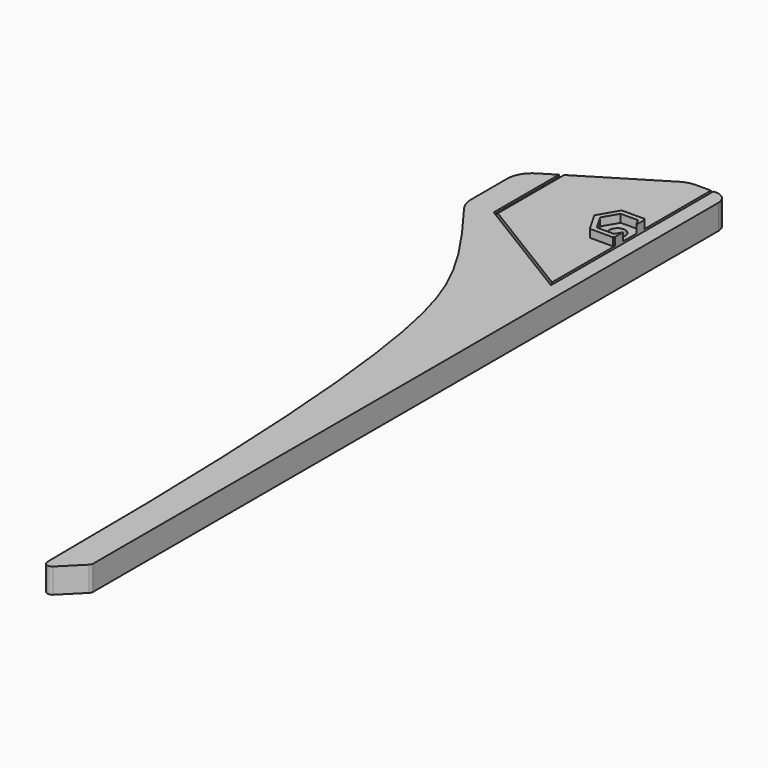
from build123d import *

# Parameters (mm, degrees)
F0_R        = 1.6
F1_DEPTH    = 2
F2_DEPTH    = 5
F3_START    = 2.1
F3_DEPTH    = 2.9
F4_SIZE     = 2.49999
F5_R        = 5
F6_R        = 2.5
F7_R        = 1
F8_START    = 2.1
F8_DEPTH    = 2.9
F9_T1_DEPTH = 29.797383518
F11_DEPTH   = 2.9
F12_DEPTH   = 4.5
F13_R       = 5


# Not quite as in the source:
# - a fillet or chamfer that OpenCascade refuses, or shapes differently, is made with other operations: its cross-section is extruded or revolved along the edge and cut away or added
# - a fillet or chamfer is up to 0.001 mm smaller than in the source, because OpenCascade refuses the exact size


with BuildPart() as f1:
    # F0 (on Top) → F1 (new body)
    with BuildSketch(Plane.XY):
        Polygon((1.5, 14.3055555556), (1.5, -2.088612395), (19, -12.7830568394), (24, -15.838612395), (24, 25), (19, 25), align=None)
        with Locations((21, 4.5806938025)):
            Circle(F0_R, mode=Mode.SUBTRACT)
        Polygon((-1, 12.7777777778), (-1, -0.5608346172), (1.5, -2.088612395), (1.5, 14.3055555556), align=None)
    extrude(amount=F1_DEPTH)

    # F0 (on Top) → F2 (join)
    with BuildSketch(Plane.XY):
        with BuildLine():
            Line((1.5, -2.088612395), (-1, -0.5608346172))
            Line((-1, -0.5608346172), (-1, 12.7777777778))
            Line((-1, 12.7777777778), (-4, 10.9444444444))
            Line((-4, 10.9444444444), (-4, -2.5923480172))
            add(Edge.make_bspline(
                [(21, -141), (21, -99.5346466722), (18.6902447603, -35.5134267653), (7.388175394, -17.5804150979), (-4, -2.5923480172)],
                knots=[0, 0, 0, 0, 0.6153681888, 1, 1, 1, 1], degree=3))
            Line((21, -141), (27, -135))
            Line((27, -135), (27, 25))
            Line((27, 25), (24, 25))
            Line((24, 25), (24, -15.838612395))
            Line((24, -15.838612395), (19, -12.7830568394))
            Line((19, -12.7830568394), (1.5, -2.088612395))
        make_face()
    extrude(amount=F2_DEPTH)

    # F0 (on Top) → F3 (join)
    with BuildSketch(Plane.XY.offset(F3_START)):
        Polygon((-1, 12.7777777778), (-1, -0.5608346172), (1.5, -2.088612395), (1.5, 14.3055555556), align=None)
    extrude(amount=F3_DEPTH)

    # F4 (size 2.5 in the source; OpenCascade refuses exactly that, so slightly less here)
    f4_edges = [f1.edges().sort_by_distance(p)[0] for p in [
        (1.5, 6.108472, 2.1),
    ]]
    chamfer(f4_edges, length=F4_SIZE)

    # F5
    f5_edges = [f1.edges().sort_by_distance(p)[0] for p in [
        (-4, 10.944444, 2.5),
        (19, 25, 1),
        (-4, -2.592348, 2.5),
    ]]
    fillet(f5_edges, radius=F5_R)

    # F6
    f6_edges = [f1.edges().sort_by_distance(p)[0] for p in [
        (27, 25, 2.5),
    ]]
    fillet(f6_edges, radius=F6_R)

    # F7
    f7_edges = [f1.edges().sort_by_distance(p)[0] for p in [
        (27, -135, 2.5),
        (21, -141, 2.5),
    ]]
    fillet(f7_edges, radius=F7_R)


with BuildPart() as f8:
    # F0 (on Top) → F8 (new body)
    with BuildSketch(Plane.XY.offset(F8_START)):
        Polygon((-1, 12.7777777778), (-1, -0.5608346172), (1.5, -2.088612395), (1.5, 14.3055555556), align=None)
        Polygon((1.5, 14.3055555556), (1.5, -2.088612395), (19, -12.7830568394), (24, -15.838612395), (24, 25), (19, 25), align=None)
        with Locations((21, 4.5806938025)):
            Circle(F0_R, mode=Mode.SUBTRACT)
    extrude(amount=F8_DEPTH)

    # F9: chamfer of 3.2 on 1 edges, made by hand

    # F9_s2 → F9_t1 (cut)
    with BuildSketch(Plane.XZ.offset(-21.0071633393)):
        Polygon((-1, 1.8), (2.2, 5), (-1, 5), align=None)
    extrude(amount=F9_T1_DEPTH, mode=Mode.SUBTRACT)

    # F10 (on face) → F11 (cut, through all)
    with BuildSketch(Plane(origin=(0, 0, 2.1), x_dir=(1, 0, 0), z_dir=(0, 0, -1))):
        Polygon((24, -1.7768462252), (24, 15.838612395), (-0.7, 0.7441679505), (-0.7, 0.1581950864), (-0.4392749953, 0.3175270337), (23.5, 14.9470839753), (23.5, -0.9108208214), align=None)
        Polygon((24, -25), (24, -7.3845413798), (23.5, -8.2505667836), (23.5, -25), align=None)
        Polygon((24, -3.7768462252), (24, -1.7768462252), (23.5, -0.9108208214), (23.5, -2.9108208214), align=None)
        Polygon((24, -7.3845413798), (24, -5.3845413798), (23.5, -6.2505667836), (23.5, -8.2505667836), align=None)
        Polygon((24, -5.3845413798), (24, -3.7768462252), (23.5, -2.9108208214), (23.5, -6.2505667836), align=None)
    extrude(amount=-F11_DEPTH, mode=Mode.SUBTRACT)

    # F10 (on face) → F12 (join)
    with BuildSketch(Plane(origin=(0, 0, 2.1), x_dir=(1, 0, 0), z_dir=(0, 0, -1))):
        Polygon((23.5, -2.9108208214), (23.5, -0.9108208214), (23.3094010768, -0.5806938025), (18.6905989232, -0.5806938025), (16.3811978465, -4.5806938025), (18.6905989232, -8.5806938025), (23.3094010768, -8.5806938025), (23.5, -8.2505667836), (23.5, -6.2505667836), (22.7320508076, -7.5806938025), (19.2679491924, -7.5806938025), (17.5358983849, -4.5806938025), (19.2679491924, -1.5806938025), (22.7320508076, -1.5806938025), align=None)
    extrude(amount=-F12_DEPTH)

    # F13
    f13_edges = [f8.edges().sort_by_distance(p)[0] for p in [
        (19, 25, 3.55),
    ]]
    fillet(f13_edges, radius=F13_R)


solid = Compound([f1.part, f8.part])
